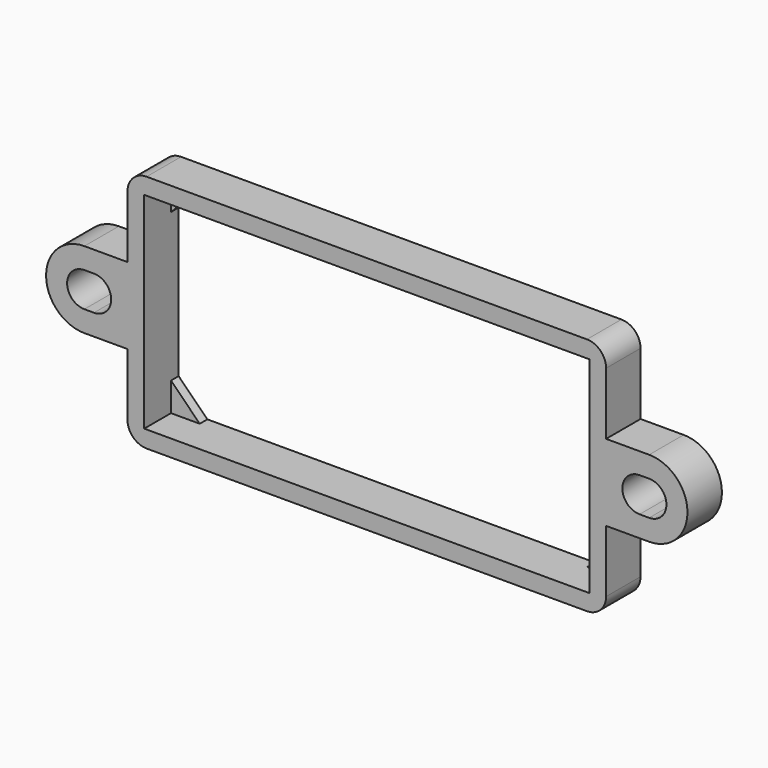
from build123d import *

# Parameters (mm, degrees)
F1_DEPTH = 4.5
F2_DEPTH = 4.501
F3_DEPTH = 1
F4_R     = 2


# Not quite as in the source:
# - a feature names something its author has since deleted; it is built from what else it names


with BuildPart() as f1:
    # F0 (on Front) → F1 (new body)
    with BuildSketch(Plane.XZ):
        Polygon((25, 12.5), (-25, 12.5), (-25, 4), (-25, -4), (-25, -12.5), (25, -12.5), (25, -4), (25, 4), align=None)
        Polygon((-23.25, 7.75), (-23.25, 10.75), (-20.25, 10.75), (20.25, 10.75), (23.25, 10.75), (23.25, 7.75), (23.25, -7.75), (23.25, -10.75), (20.25, -10.75), (-20.25, -10.75), (-23.25, -10.75), (-23.25, -7.75), align=None, mode=Mode.SUBTRACT)
        Polygon((-20.25, 10.75), (-23.25, 10.75), (-23.25, 7.75), align=None)
        Polygon((23.25, 10.75), (20.25, 10.75), (23.25, 7.75), align=None)
        with BuildLine():
            Line((-25, -4), (-25, 4))
            Line((-25, 4), (-29.5, 4))
            ThreePointArc((-29.5, 4), (-33.5, 0), (-29.5, -4))
            Line((-29.5, -4), (-25, -4))
        make_face()
        with BuildLine():
            Line((-28.5, -1.8), (-29.5, -1.8))
            ThreePointArc((-29.5, -1.8), (-31.3, 0), (-29.5, 1.8))
            Line((-29.5, 1.8), (-28.5, 1.8))
            ThreePointArc((-28.5, 1.8), (-26.7, 0), (-28.5, -1.8))
        make_face(mode=Mode.SUBTRACT)
        with BuildLine():
            Line((29.5, 4), (25, 4))
            Line((25, 4), (25, -4))
            Line((25, -4), (29.5, -4))
            ThreePointArc((29.5, -4), (33.5, 0), (29.5, 4))
        make_face()
        with BuildLine():
            ThreePointArc((29.5, 1.8), (31.3, 0), (29.5, -1.8))
            Line((29.5, -1.8), (28.5, -1.8))
            ThreePointArc((28.5, -1.8), (26.7, 0), (28.5, 1.8))
            Line((28.5, 1.8), (29.5, 1.8))
        make_face(mode=Mode.SUBTRACT)
    extrude(amount=F1_DEPTH)

    # F0 (on Front) → F2 (cut, through all)
    with BuildSketch(Plane.XZ):
        Polygon((-20.25, 10.75), (-23.25, 10.75), (-23.25, 7.75), align=None)
        Polygon((20.25, 10.75), (-20.25, 10.75), (-23.25, 7.75), (-23.25, -7.75), (-20.25, -10.75), (20.25, -10.75), (23.25, -7.75), (23.25, 7.75), align=None)
        Polygon((23.25, 10.75), (20.25, 10.75), (23.25, 7.75), align=None)
    extrude(amount=F2_DEPTH, mode=Mode.SUBTRACT)

    # F0 (on Front) → F3 (join)
    with BuildSketch(Plane.XZ):
        Polygon((23.25, 10.75), (20.25, 10.75), (23.25, 7.75), align=None)
        Polygon((23.25, -10.75), (23.25, -7.75), (20.25, -10.75), align=None)
        Polygon((-20.25, 10.75), (-23.25, 10.75), (-23.25, 7.75), align=None)
        Polygon((-20.25, -10.75), (-23.25, -7.75), (-23.25, -10.75), align=None)
    extrude(amount=F3_DEPTH)

    # F4
    f4_edges = [f1.edges().sort_by_distance(p)[0] for p in [
        (-25, -2.25, -12.5),
        (25, -2.25, -12.5),
        (25, -2.25, 12.5),
        (-25, -2.25, 12.5),
    ]]
    fillet(f4_edges, radius=F4_R)


solid = f1.part
